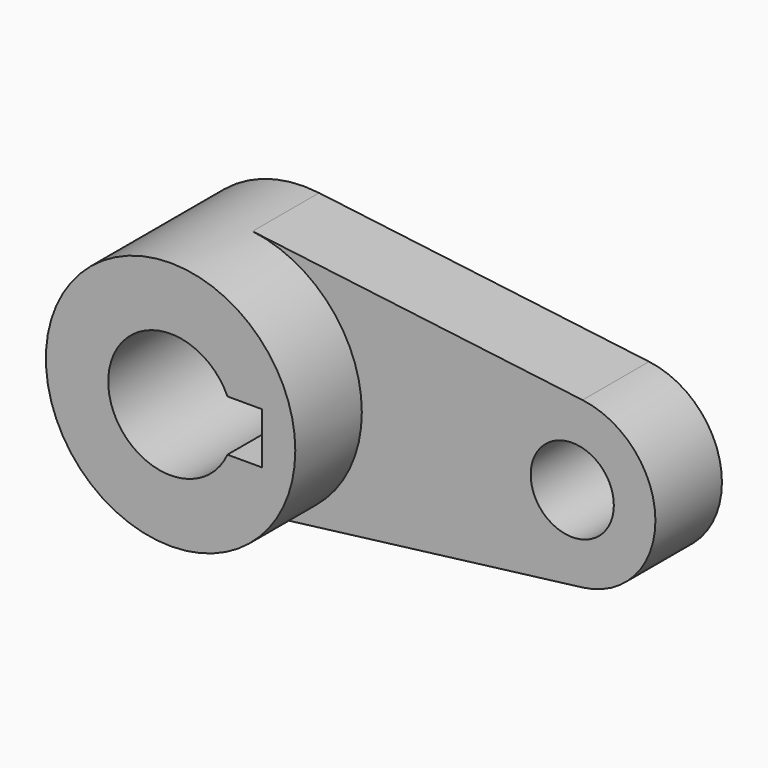
from build123d import *

# Parameters (mm, degrees)
F0_R     = 12.7
F1_DEPTH = 25.4
F2_DEPTH = 50.8


# Not quite as in the source:
# - a feature names something its author has since deleted; it is built from what else it names


with BuildPart() as f1:
    # F0 (on Front) → F1 (new body)
    with BuildSketch(Plane.XZ):
        with BuildLine():
            ThreePointArc((4.7257233878, 37.8057871028), (28.5627384986, 25.2146776593), (38.1, 0))
            ThreePointArc((38.1, 0), (28.5627384986, -25.2146776593), (4.7257233878, -37.8057871028))
            Line((4.7257233878, -37.8057871028), (105.541155662, -25.2038580685))
            ThreePointArc((105.541155662, -25.2038580685), (76.9906734034, 0), (105.541155662, 25.2038580685))
            Line((105.541155662, 25.2038580685), (4.7257233878, 37.8057871028))
        make_face()
        with BuildLine():
            ThreePointArc((127.7906734034, 0), (121.4324990691, 16.8097851062), (105.541155662, 25.2038580685))
            ThreePointArc((105.541155662, 25.2038580685), (76.9906734034, 0), (105.541155662, -25.2038580685))
            ThreePointArc((105.541155662, -25.2038580685), (121.4324990691, -16.8097851062), (127.7906734034, 0))
        make_face()
        with Locations((102.3906734034, 0)):
            Circle(F0_R, mode=Mode.SUBTRACT)
        with BuildLine():
            ThreePointArc((4.7257233878, -37.8057871028), (28.5627384986, -25.2146776593), (38.1, 0))
            ThreePointArc((38.1, 0), (28.5627384986, 25.2146776593), (4.7257233878, 37.8057871028))
            ThreePointArc((4.7257233878, 37.8057871028), (-38.1, 0), (4.7257233878, -37.8057871028))
        make_face()
        with BuildLine():
            ThreePointArc((-17.3665807845, 7.8297108412), (0, 19.05), (17.3665807845, 7.8297108412))
            Line((17.3665807845, 7.8297108412), (27.8837817341, 7.8297108412))
            Line((27.8837817341, 7.8297108412), (27.8837817341, -7.8297108412))
            Line((27.8837817341, -7.8297108412), (17.3665807845, -7.8297108412))
            ThreePointArc((17.3665807845, -7.8297108412), (0, -19.05), (-17.3665807845, -7.8297108412))
            Line((-17.3665807845, -7.8297108412), (-22.9162182659, -7.8297108412))
            Line((-22.9162182659, -7.8297108412), (-22.9162182659, 0))
            Line((-22.9162182659, 0), (-22.9162182659, 7.8297108412))
            Line((-22.9162182659, 7.8297108412), (-17.3665807845, 7.8297108412))
        make_face(mode=Mode.SUBTRACT)
        with BuildLine():
            ThreePointArc((-17.3665807845, -7.8297108412), (-19.05, 0), (-17.3665807845, 7.8297108412))
            Line((-17.3665807845, 7.8297108412), (-22.9162182659, 7.8297108412))
            Line((-22.9162182659, 7.8297108412), (-22.9162182659, 0))
            Line((-22.9162182659, 0), (-22.9162182659, -7.8297108412))
            Line((-22.9162182659, -7.8297108412), (-17.3665807845, -7.8297108412))
        make_face()
    extrude(amount=F1_DEPTH)

    # F0 (on Front) → F2 (join)
    with BuildSketch(Plane.XZ):
        with BuildLine():
            ThreePointArc((4.7257233878, -37.8057871028), (28.5627384986, -25.2146776593), (38.1, 0))
            ThreePointArc((38.1, 0), (28.5627384986, 25.2146776593), (4.7257233878, 37.8057871028))
            ThreePointArc((4.7257233878, 37.8057871028), (-38.1, 0), (4.7257233878, -37.8057871028))
        make_face()
        with BuildLine():
            ThreePointArc((-17.3665807845, 7.8297108412), (0, 19.05), (17.3665807845, 7.8297108412))
            Line((17.3665807845, 7.8297108412), (27.8837817341, 7.8297108412))
            Line((27.8837817341, 7.8297108412), (27.8837817341, -7.8297108412))
            Line((27.8837817341, -7.8297108412), (17.3665807845, -7.8297108412))
            ThreePointArc((17.3665807845, -7.8297108412), (0, -19.05), (-17.3665807845, -7.8297108412))
            Line((-17.3665807845, -7.8297108412), (-22.9162182659, -7.8297108412))
            Line((-22.9162182659, -7.8297108412), (-22.9162182659, 0))
            Line((-22.9162182659, 0), (-22.9162182659, 7.8297108412))
            Line((-22.9162182659, 7.8297108412), (-17.3665807845, 7.8297108412))
        make_face(mode=Mode.SUBTRACT)
        with BuildLine():
            ThreePointArc((-17.3665807845, -7.8297108412), (-19.05, 0), (-17.3665807845, 7.8297108412))
            Line((-17.3665807845, 7.8297108412), (-22.9162182659, 7.8297108412))
            Line((-22.9162182659, 7.8297108412), (-22.9162182659, 0))
            Line((-22.9162182659, 0), (-22.9162182659, -7.8297108412))
            Line((-22.9162182659, -7.8297108412), (-17.3665807845, -7.8297108412))
        make_face()
    extrude(amount=F2_DEPTH)


solid = f1.part
